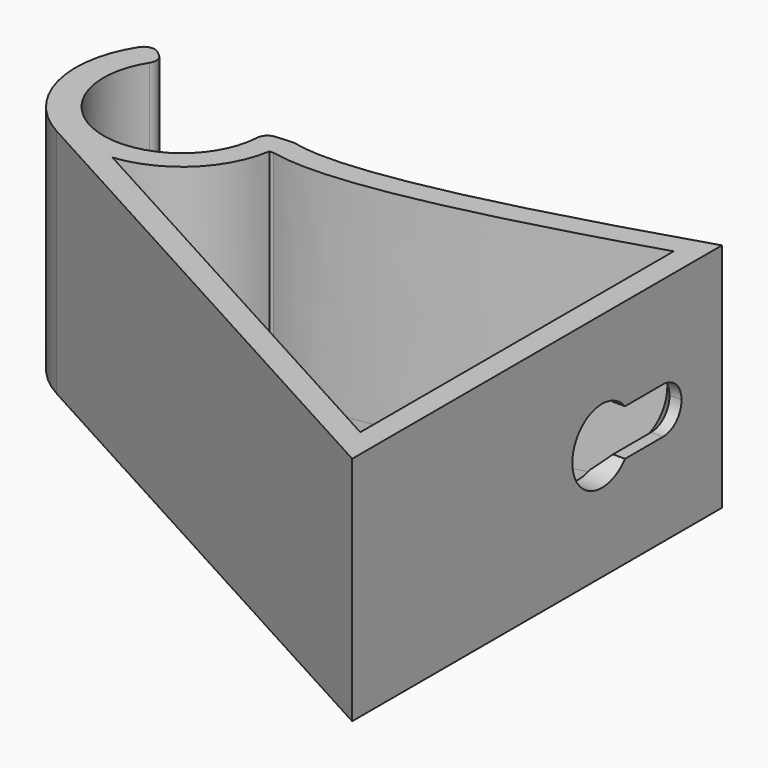
from build123d import *

# Parameters (mm, degrees)
F1_DEPTH = 25
F2_R     = 1.2
F3_T     = -2.5
F4_DEPTH = 25
F6_DEPTH = 3
F7_SIZE  = 1.2


with BuildPart() as f1:
    # F0 (on Top) → F1 (new body)
    with BuildSketch(Plane.XY):
        with BuildLine():
            Line((0, -23.9775525033), (0, 0))
            Line((0, 0), (0, 26.0224474967))
            add(Edge.make_bspline(
                [(0, 26.0224474967), (-17.6971325381, 20.4363816506), (-33.2169395037, 16.3747998881), (-39.9791178567, 18.1051199008)],
                knots=[0, 0, 0, 0, 0.723504363, 0.723504363, 0.723504363, 0.723504363], degree=3))
            ThreePointArc((-39.9791178567, 18.1051199008), (-45.2661850168, 7.6441593667), (-56.9807893445, 7.2532375123))
            Line((-56.9807893445, 7.2532375123), (0, -23.9775525033))
        make_face()
        with BuildLine():
            ThreePointArc((-56.9807893445, 7.2532375123), (-45.2661850168, 7.6441593667), (-39.9791178567, 18.1051199008))
            Line((-39.9791178567, 18.1051199008), (-42.9724328811, 17.9049570556))
            ThreePointArc((-42.9724328811, 17.9049570556), (-54.0664587009, 9.2494171829), (-57.9998429251, 22.7595714353))
            Line((-57.9998429251, 22.7595714353), (-60.310319681, 24.6731275909))
            ThreePointArc((-60.310319681, 24.6731275909), (-62.749017961, 15.17887186), (-56.9807893445, 7.2532375123))
        make_face()
    extrude(amount=F1_DEPTH)

    # F2
    f2_edges = [f1.edges().sort_by_distance(p)[0] for p in [
        (-57.999843, 22.759571, 12.5),
        (-60.31032, 24.673128, 12.5),
        (-42.972433, 17.904957, 12.5),
    ]]
    fillet(f2_edges, radius=F2_R)

    # F3
    f3_openings = [f1.faces().sort_by_distance(p)[0] for p in [
        (-21.146453, 4.166771, 25),
    ]]
    offset(amount=F3_T, openings=f3_openings)

    # F4 (cut): a face of the model
    f4_faces = [f1.faces().sort_by_distance(p)[0] for p in [
        (-19.3393150943, 3.8306877566, 2.5),
    ]]
    extrude(f4_faces, amount=-F4_DEPTH, mode=Mode.SUBTRACT)

    # F5 (on face) → F6 (cut)
    with BuildSketch(Plane.YZ):
        with BuildLine():
            ThreePointArc((12.9166145043, 10), (13.5683701333, 11.1752351146), (13.7941155051, 12.5))
            ThreePointArc((13.7941155051, 12.5), (13.5683701333, 13.8247648854), (12.9166145043, 15))
            ThreePointArc((12.9166145043, 15), (5.7941155051, 12.5), (12.9166145043, 10))
        make_face()
        with BuildLine():
            ThreePointArc((20.5641841143, 12.5), (19.8319510673, 14.267766953), (18.0641841143, 15))
            ThreePointArc((18.0641841143, 15), (15.5641841143, 12.5), (18.0641841143, 10))
            ThreePointArc((18.0641841143, 10), (19.8319510673, 10.732233047), (20.5641841143, 12.5))
        make_face()
        with BuildLine():
            ThreePointArc((12.9166145043, 15), (13.5683701333, 13.8247648854), (13.7941155051, 12.5))
            ThreePointArc((13.7941155051, 12.5), (13.5683701333, 11.1752351146), (12.9166145043, 10))
            Line((12.9166145043, 10), (18.0641841143, 10))
            ThreePointArc((18.0641841143, 10), (15.5641841143, 12.5), (18.0641841143, 15))
            Line((18.0641841143, 15), (12.9166145043, 15))
        make_face()
    extrude(amount=-F6_DEPTH, mode=Mode.SUBTRACT)

    # F7
    f7_edges = [f1.edges().sort_by_distance(p)[0] for p in [
        (-2.5, 15.490399, 10),
        (-2.5, 15.490399, 15),
        (-2.5, 20.564184, 12.5),
    ]]
    chamfer(f7_edges, length=F7_SIZE)


solid = f1.part
